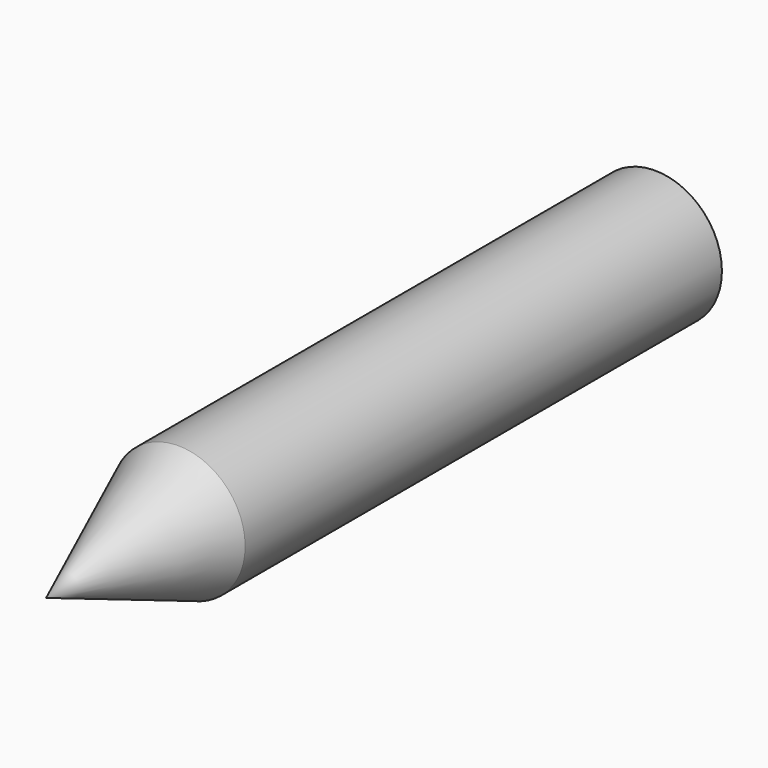
from build123d import *

# Parameters (mm, degrees)
F0_R     = 17.0815
F0_R_2   = 12.7
F1_DEPTH = 152.4
F2_R     = 17.0815


# Not quite as in the source:
# - an extrude whose draft closes it to a point is written as a loft to that point


with BuildPart() as f1:
    # F0 (on Front) → F1 (new body)
    with BuildSketch(Plane.XZ):
        Circle(F0_R)
        Circle(F0_R_2, mode=Mode.SUBTRACT)
    extrude(amount=F1_DEPTH)

    # F2 (on face) → F3 section 0
    with BuildSketch(Plane.XZ.offset(152.4), mode=Mode.PRIVATE) as f3_s0:
        Circle(F2_R)
    loft([f3_s0.sketch, Vertex(0, -194.6781960866, 0)], ruled=True)


solid = f1.part
